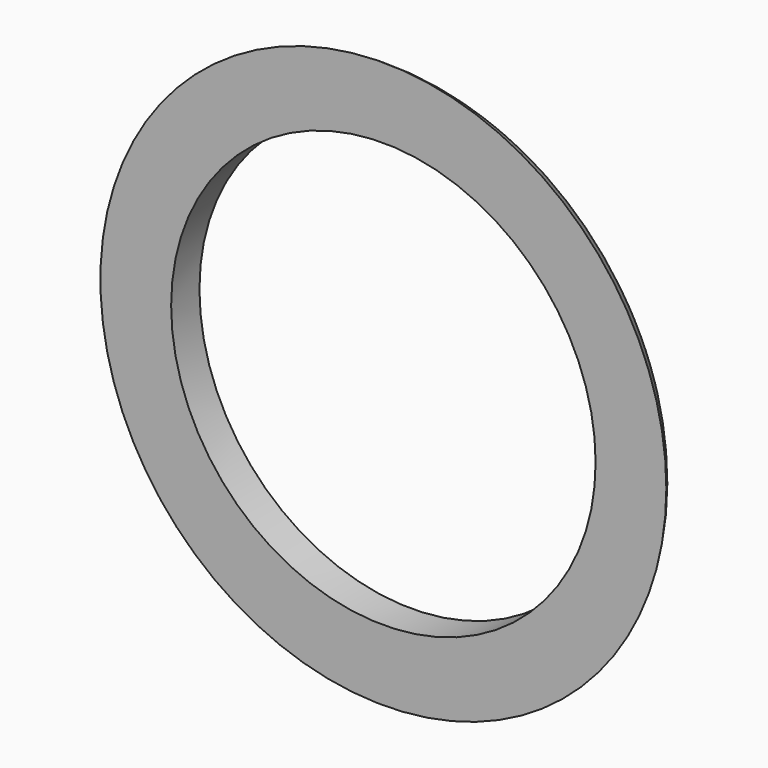
from build123d import *

# Parameters (mm, degrees)
F0_R     = 20
F0_R_2   = 15
F1_DEPTH = 2.5


# Not quite as in the source:
# - a fillet or chamfer that OpenCascade refuses, or shapes differently, is made with other operations: its cross-section is extruded or revolved along the edge and cut away or added


with BuildPart() as f1:
    # F0 (on Front) → F1 (new body)
    with BuildSketch(Plane.XZ):
        Circle(F0_R)
        Circle(F0_R_2, mode=Mode.SUBTRACT)
    extrude(amount=F1_DEPTH)

    # F2: fillet of radius 5 on 1 edges, made by hand

    # F2_s1 → F2_t2 (revolve, cut)
    with BuildSketch(Plane.XY):
        with BuildLine():
            ThreePointArc((20, -2.5), (18.1698729811, -0.6698729811), (15.6698729811, 0))
            Line((15.6698729811, 0), (20, 0))
            Line((20, 0), (20, -2.5))
        make_face()
    revolve(axis=Axis((0, 0, 0), (0, -1, 0)), mode=Mode.SUBTRACT)


solid = f1.part
